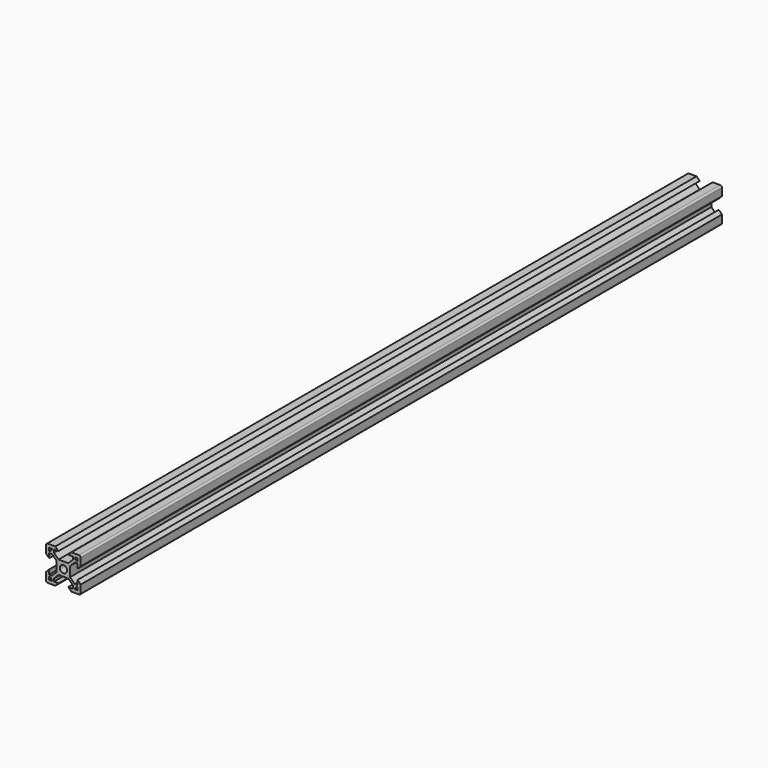
from build123d import *

# Parameters (mm, degrees)
F0_W            = 20
F0_H            = 20
F1_DEPTH        = 463
F2_R            = 2.1
F3_DEPTH        = 463.001
F4_R            = 1
F6_DEPTH        = 463.001
F6_COPIES_COUNT = 4


# Not quite as in the source:
# - a pattern or mirror of a feature is missing from the dataset's text; its kind, count and spacing are read off the source's solid


with BuildPart() as f1:
    # F0 (on Front) → F1 (new body)
    with BuildSketch(Plane.XZ):
        Rectangle(F0_W, F0_H)
    extrude(amount=F1_DEPTH)

    # F2 (on face) → F3 (cut, through all)
    with BuildSketch(Plane.XZ.offset(463)):
        Circle(F2_R)
    extrude(amount=-F3_DEPTH, mode=Mode.SUBTRACT)

    # F4
    f4_edges = [f1.edges().sort_by_distance(p)[0] for p in [
        (-10, -231.5, 10),
        (10, -231.5, 10),
        (10, -231.5, -10),
        (-10, -231.5, -10),
    ]]
    fillet(f4_edges, radius=F4_R)

    # F5 (on face) → F6 (cut, through all)
    with BuildSketch(Plane.XZ.offset(463)):
        Polygon((0, 3.9006601718), (0, 10), (-2.84, 10), (-4.64, 10), (-2.84, 8.2), (-5.4993398282, 8.2), (-5.4993398282, 6.56), (-2.84, 3.9006601718), align=None)
        Polygon((-6.5693398282, 8.2), (-8.2, 8.2), (-7.0953059148, 7.0953059148), (-6.5693398282, 7.6212720014), align=None)
    f6 = extrude(amount=-F6_DEPTH, mode=Mode.SUBTRACT)

    # F6_copies: F6 ×4 about axis
    f6_copies_axis = Axis((0, 0, 0), (0, 1, 0))
    for i in range(1, F6_COPIES_COUNT):
        add(f6.rotate(f6_copies_axis, i * 360 / F6_COPIES_COUNT), mode=Mode.SUBTRACT)

    # F6_copies1: F6 across plane
    add(f6.mirror(Plane(origin=(0, 0, 0), x_dir=(-0.7071067812, 0, -0.7071067812), z_dir=(0.7071067812, 0, -0.7071067812))), mode=Mode.SUBTRACT)

    # F6_copies2: F6 across plane
    add(f6.mirror(Plane(origin=(0, 0, 0), x_dir=(-1, 0, 0), z_dir=(0, 0, -1))), mode=Mode.SUBTRACT)

    # F6_copies3: F6 across plane
    add(f6.mirror(Plane(origin=(0, 0, 0), x_dir=(0, 0, 1), z_dir=(1, 0, 0))), mode=Mode.SUBTRACT)

    # F6_copies4: F6 across plane
    add(f6.mirror(Plane(origin=(0, 0, 0), x_dir=(0.7071067812, 0, -0.7071067812), z_dir=(-0.7071067812, 0, -0.7071067812))), mode=Mode.SUBTRACT)


solid = f1.part
